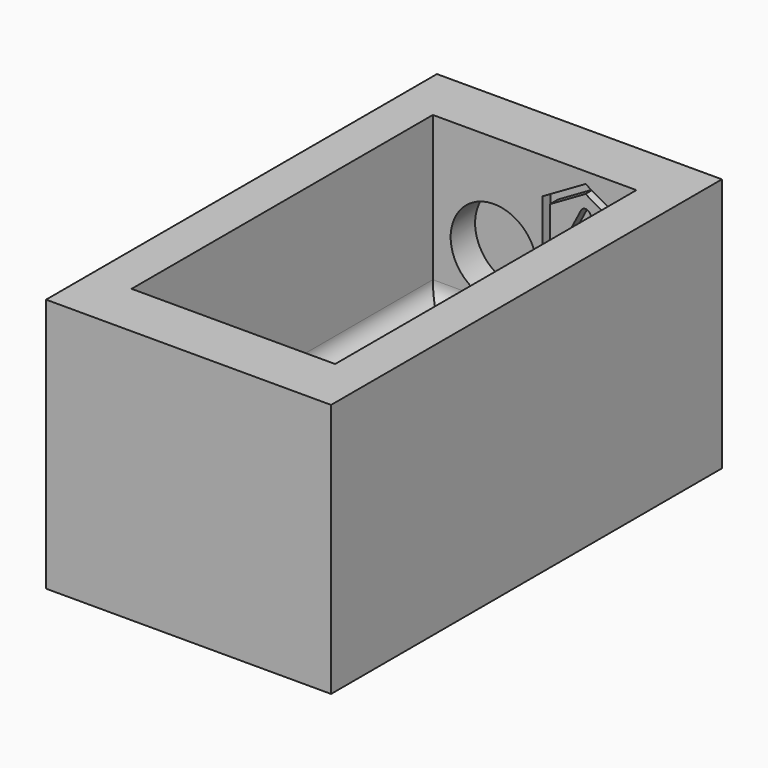
from build123d import *

# Parameters (mm, degrees)
F0_W      = 28
F0_H      = 48
F1_DEPTH  = 25
F2_W      = 20
F2_H      = 37
F3_DEPTH  = 16
F4_R      = 3
F4_R_2    = 1.575
F5_DEPTH  = 2
F6_R      = 5
F6_R_2    = 3
F7_DEPTH  = 4
F9_DEPTH  = 9.001
F10_R     = 4.25
F11_DEPTH = 3
F13_DEPTH = 1
F17_DEPTH = 1
F18_R     = 1.74999


# Not quite as in the source:
# - a fillet or chamfer is up to 0.001 mm smaller than in the source, because OpenCascade refuses the exact size


with BuildPart() as f1:
    # F0 (on Top) → F1 (new body)
    with BuildSketch(Plane.XY):
        with Locations((-14, 24)):
            Rectangle(F0_W, F0_H)
    extrude(amount=F1_DEPTH)

    # F2 (on face) → F3 (cut)
    with BuildSketch(Plane.XY.offset(25)):
        with Locations((-14, 24)):
            Rectangle(F2_W, F2_H)
    extrude(amount=-F3_DEPTH, mode=Mode.SUBTRACT)

    # F4 (on face) → F5 (join)
    with BuildSketch(Plane.XY.offset(9)):
        with Locations((-11, 24)):
            Circle(F4_R)
        with Locations((-11, 24)):
            Circle(F4_R_2, mode=Mode.SUBTRACT)
    extrude(amount=F5_DEPTH)

    # F6 (on face) → F7 (cut)
    with BuildSketch(Plane.XY.offset(9)):
        with Locations((-11, 24)):
            Circle(F6_R)
        with Locations((-11, 24)):
            Circle(F6_R_2, mode=Mode.SUBTRACT)
    extrude(amount=-F7_DEPTH, mode=Mode.SUBTRACT)

    # F9 (cut, through all): a face of the model
    f9_faces = [f1.faces().sort_by_distance(p)[0] for p in [
        (-11, 24, 9),
    ]]
    extrude(f9_faces, amount=-F9_DEPTH, mode=Mode.SUBTRACT)

    # F10 (on face) → F11 (cut)
    with BuildSketch(Plane.XZ.offset(-42.5)):
        with Locations((-18, 15)):
            Circle(F10_R)
    extrude(amount=-F11_DEPTH, mode=Mode.SUBTRACT)

    # F12 (on face) → F13 (cut)
    with BuildSketch(Plane(origin=(0, 48, 0), x_dir=(-1, 0, 0), z_dir=(0, 1, 0))):
        with BuildLine():
            ThreePointArc((11, 20), (10.2928932188, 19.7071067812), (10, 19))
            Line((10, 19), (10, 7))
            ThreePointArc((10, 7), (10.2928932188, 6.2928932188), (11, 6))
            Line((11, 6), (17, 6))
            ThreePointArc((17, 6), (17.7071067812, 6.2928932188), (18, 7))
            ThreePointArc((18, 7), (17.7071067812, 7.7071067812), (17, 8))
            Line((17, 8), (12.5, 8))
            ThreePointArc((12.5, 8), (12.1464466094, 8.1464466094), (12, 8.5))
            Line((12, 8.5), (12, 19))
            ThreePointArc((12, 19), (11.7071067812, 19.7071067812), (11, 20))
        make_face()
    extrude(amount=-F13_DEPTH, mode=Mode.SUBTRACT)

    # F15 (on face) → F17 (cut)
    with BuildSketch(Plane.XZ.offset(-42.5)):
        Polygon((-9, 14.0925227119), (-4.75, 16.5462613559), (-4.75, 21.4537386441), (-9, 23.9074772881), (-13.25, 21.4537386441), (-13.25, 16.5462613559), align=None)
        Polygon((-9, 14.9585481157), (-12.5, 16.9792740578), (-12.5, 21.0207259422), (-9, 23.0414518843), (-5.5, 21.0207259422), (-5.5, 16.9792740578), align=None, mode=Mode.SUBTRACT)
        with BuildLine():
            Line((-10.4970194787, 17.2914120527), (-11.3840303118, 17.7531606659))
            ThreePointArc((-11.3840303118, 17.7531606659), (-11.1713992019, 17.0787809427), (-10.4970194787, 17.2914120527))
        make_face()
        with BuildLine():
            ThreePointArc((-9.4435054166, 21.0191256934), (-9.5, 21.25), (-9.4435054166, 21.4808743066))
            Line((-9.4435054166, 21.4808743066), (-11.3840303118, 17.7531606659))
            Line((-11.3840303118, 17.7531606659), (-10.4970194787, 17.2914120527))
            Line((-10.4970194787, 17.2914120527), (-9, 20.1671597149))
            Line((-9, 20.1671597149), (-9.4435054166, 21.0191256934))
        make_face()
        with BuildLine():
            ThreePointArc((-8.5564945834, 21.0191256934), (-8.5143289651, 21.1311570538), (-8.5, 21.25))
            ThreePointArc((-8.5, 21.25), (-8.5143289651, 21.3688429462), (-8.5564945834, 21.4808743066))
            ThreePointArc((-8.5564945834, 21.4808743066), (-9, 21.75), (-9.4435054166, 21.4808743066))
            ThreePointArc((-9.4435054166, 21.4808743066), (-9.5, 21.25), (-9.4435054166, 21.0191256934))
            ThreePointArc((-9.4435054166, 21.0191256934), (-9, 20.75), (-8.5564945834, 21.0191256934))
        make_face()
        with BuildLine():
            Line((-9, 20.1671597149), (-8.5564945834, 21.0191256934))
            ThreePointArc((-8.5564945834, 21.0191256934), (-9, 20.75), (-9.4435054166, 21.0191256934))
            Line((-9.4435054166, 21.0191256934), (-9, 20.1671597149))
        make_face()
        with BuildLine():
            ThreePointArc((-8.5564945834, 21.4808743066), (-8.5143289651, 21.3688429462), (-8.5, 21.25))
            ThreePointArc((-8.5, 21.25), (-8.5143289651, 21.1311570538), (-8.5564945834, 21.0191256934))
            Line((-8.5564945834, 21.0191256934), (-9, 20.1671597149))
            Line((-9, 20.1671597149), (-7.5029805213, 17.2914120527))
            Line((-7.5029805213, 17.2914120527), (-6.6159696882, 17.7531606659))
            Line((-6.6159696882, 17.7531606659), (-8.5564945834, 21.4808743066))
        make_face()
        with BuildLine():
            ThreePointArc((-7.5029805213, 17.2914120527), (-6.8286007981, 17.0787809427), (-6.6159696882, 17.7531606659))
            Line((-6.6159696882, 17.7531606659), (-7.5029805213, 17.2914120527))
        make_face()
    extrude(amount=-F17_DEPTH, mode=Mode.SUBTRACT)

    # F18 (radius 1.75 in the source; OpenCascade refuses exactly that, so slightly less here)
    f18_edges = [f1.edges().sort_by_distance(p)[0] for p in [
        (-24, 24, 9),
        (-14, 42.5, 9),
        (-4, 24, 9),
        (-14, 5.5, 9),
    ]]
    fillet(f18_edges, radius=F18_R)


solid = f1.part
